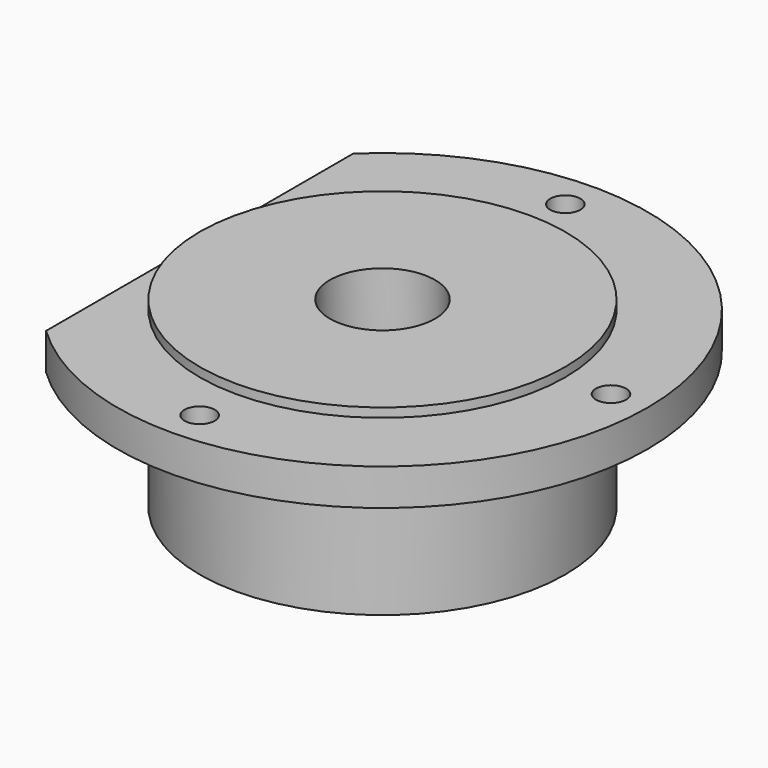
from build123d import *

# Parameters (mm, degrees)
F3_D     = 6.6
F5_DEPTH = 25


# Not quite as in the source:
# - a feature names something its author has since deleted; it is built from what else it names


with BuildPart() as f1:
    # F0 (on Right) → F1 (revolve)
    with BuildSketch(Plane.YZ):
        Polygon((-11.5, 40), (-40, 40), (-40, 38), (-58, 38), (-58, 30), (-40, 30), (-40, 0), (-30, 0), (-30, 28), (-11.5, 28), align=None)
    revolve(axis=Axis((0, 0, 32.5555), (0, 0, 1)))

    # F3 (through all)
    with Locations(Plane.XY.offset(40)):
        with Locations((-50, 0), (0, 50), (50, 0), (0, -50)):
            Hole(F3_D / 2)

    # F4 (on face) → F5 (cut)
    with BuildSketch(Plane.XY.offset(38)):
        with BuildLine():
            Line((-40, -42), (-40, 0))
            Line((-40, 0), (-46.7, 0))
            ThreePointArc((-46.7, 0), (-50, -3.3), (-53.3, 0))
            Line((-53.3, 0), (-58, 0))
            ThreePointArc((-58, 0), (-53.310411741, -22.8473193176), (-40, -42))
        make_face()
        with BuildLine():
            Line((-46.7, 0), (-40, 0))
            Line((-40, 0), (-40, 42))
            ThreePointArc((-40, 42), (-53.310411741, 22.8473193176), (-58, 0))
            Line((-58, 0), (-53.3, 0))
            ThreePointArc((-53.3, 0), (-50, 3.3), (-46.7, 0))
        make_face()
        with BuildLine():
            Line((-40, -44.474773109), (-40, -42))
            ThreePointArc((-40, -42), (-53.310411741, -22.8473193176), (-58, 0))
            Line((-58, 0), (-66.5342658758, 0))
            Line((-66.5342658758, 0), (-66.5342658758, -44.474773109))
            Line((-66.5342658758, -44.474773109), (-40, -44.474773109))
        make_face()
        with BuildLine():
            ThreePointArc((-58, 0), (-53.310411741, 22.8473193176), (-40, 42))
            Line((-40, 42), (-40, 51.5907406807))
            Line((-40, 51.5907406807), (-66.5342658758, 51.5907406807))
            Line((-66.5342658758, 51.5907406807), (-66.5342658758, 0))
            Line((-66.5342658758, 0), (-58, 0))
        make_face()
    extrude(amount=-F5_DEPTH, mode=Mode.SUBTRACT)


solid = f1.part
